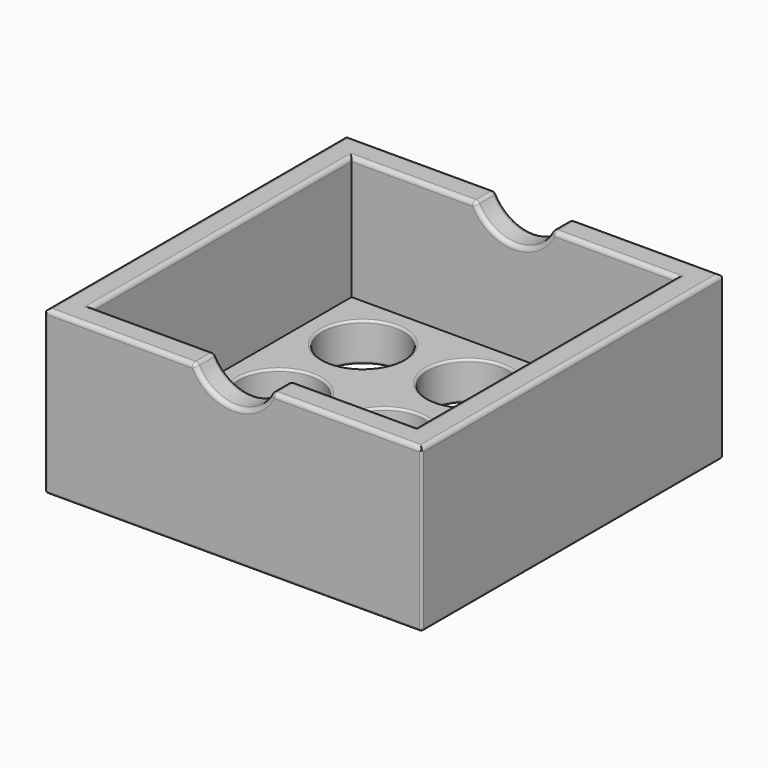
from build123d import *

# Parameters (mm, degrees)
F0_W         = 74
F0_H         = 74
F1_DEPTH     = 37
F0_R         = 9.25
F2_DEPTH     = 8.8
F3_R         = 9.6387493407
F4_DEPTH     = 800
F5_R         = 1
F6_T1_DEPTH  = 36.75
F6_T3_DEPTH  = 85
F6_T5_DEPTH  = 85
F6_S9_W      = 0.51
F6_S9_H      = 0.51
F6_T10_DEPTH = 0.51
F6_S15_W     = 0.51
F6_S15_H     = 0.51
F6_T16_DEPTH = 0.51
F6_S21_W     = 0.51
F6_S21_H     = 0.51
F6_T22_DEPTH = 0.51
F6_S27_W     = 0.51
F6_S27_H     = 0.51
F6_T28_DEPTH = 0.51
F7_R         = 0.5


# Not quite as in the source:
# - a fillet or chamfer that OpenCascade refuses, or shapes differently, is made with other operations: its cross-section is extruded or revolved along the edge and cut away or added


with BuildPart() as f1:
    # F0 (on Top) → F1 (new body)
    with BuildSketch(Plane.XY):
        Polygon((-6, 80), (-6, 0), (-6, -6), (80, -6), (80, 80), align=None)
        with Locations((37, 37)):
            Rectangle(F0_W, F0_H, mode=Mode.SUBTRACT)
    extrude(amount=F1_DEPTH)

    # F0 (on Top) → F2 (join)
    with BuildSketch(Plane.XY):
        with Locations((37, 37)):
            Rectangle(F0_W, F0_H)
        with Locations((13, 13)):
            Circle(F0_R, mode=Mode.SUBTRACT)
        with Locations((37, 13)):
            Circle(F0_R, mode=Mode.SUBTRACT)
        with Locations((61, 13)):
            Circle(F0_R, mode=Mode.SUBTRACT)
        with Locations((13, 37)):
            Circle(F0_R, mode=Mode.SUBTRACT)
        with Locations((13, 61)):
            Circle(F0_R, mode=Mode.SUBTRACT)
        with Locations((37, 37)):
            Circle(F0_R, mode=Mode.SUBTRACT)
        with Locations((61, 37)):
            Circle(F0_R, mode=Mode.SUBTRACT)
        with Locations((37, 61)):
            Circle(F0_R, mode=Mode.SUBTRACT)
        with Locations((61, 61)):
            Circle(F0_R, mode=Mode.SUBTRACT)
    extrude(amount=F2_DEPTH)

    # F3 (on face) → F4 (cut)
    with BuildSketch(Plane.XZ.offset(6)):
        with Locations((37, 41)):
            Circle(F3_R)
    extrude(amount=-F4_DEPTH, mode=Mode.SUBTRACT)

    # F5
    f5_edges = [f1.edges().sort_by_distance(p)[0] for p in [
        (-6, 37, 37),
        (11.115211, 80, 37),
        (28.230423, 77, 37),
        (14.115211, 74, 37),
        (0, 37, 37),
        (14.115211, 0, 37),
        (28.230423, -3, 37),
        (11.115211, -6, 37),
        (62.884789, -6, 37),
        (45.769577, -3, 37),
        (59.884789, 0, 37),
        (74, 37, 37),
        (59.884789, 74, 37),
        (45.769577, 77, 37),
        (62.884789, 80, 37),
        (80, 37, 37),
        (37, -6, 31.361251),
        (37, 0, 31.361251),
        (37, 74, 31.361251),
        (37, 80, 31.361251),
    ]]
    fillet(f5_edges, radius=F5_R)

    # F6: fillet of radius 0.5 on 16 edges, made by hand

    # F6_s2 → F6_t1 (cut)
    with BuildSketch(Plane.XY.offset(0.5)):
        with BuildLine():
            ThreePointArc((79.5, -6), (79.8535533906, -5.8535533906), (80, -5.5))
            Line((80, -5.5), (80, -6))
            Line((80, -6), (79.5, -6))
        make_face()
        with BuildLine():
            ThreePointArc((-6, -5.5), (-5.8535533906, -5.8535533906), (-5.5, -6))
            Line((-5.5, -6), (-6, -6))
            Line((-6, -6), (-6, -5.5))
        make_face()
        with BuildLine():
            ThreePointArc((79.5, 80), (79.8535533906, 79.8535533906), (80, 79.5))
            Line((80, 79.5), (80, 80))
            Line((80, 80), (79.5, 80))
        make_face()
        with BuildLine():
            ThreePointArc((-6, 79.5), (-5.8535533906, 79.8535533906), (-5.5, 80))
            Line((-5.5, 80), (-6, 80))
            Line((-6, 80), (-6, 79.5))
        make_face()
    extrude(amount=F6_T1_DEPTH, mode=Mode.SUBTRACT)

    # F6_s4 → F6_t3 (cut)
    with BuildSketch(Plane.YZ.offset(-5.5)):
        with BuildLine():
            ThreePointArc((-5.5, 0), (-5.8535533906, 0.1464466094), (-6, 0.5))
            Line((-6, 0.5), (-6, 0))
            Line((-6, 0), (-5.5, 0))
        make_face()
        with BuildLine():
            ThreePointArc((80, 0.5), (79.8535533906, 0.1464466094), (79.5, 0))
            Line((79.5, 0), (80, 0))
            Line((80, 0), (80, 0.5))
        make_face()
    extrude(amount=F6_T3_DEPTH, mode=Mode.SUBTRACT)

    # F6_s6 → F6_t5 (cut)
    with BuildSketch(Plane.XZ.offset(-79.5)):
        with BuildLine():
            ThreePointArc((79.5, 0), (79.8535533906, 0.1464466094), (80, 0.5))
            Line((80, 0.5), (80, 0))
            Line((80, 0), (79.5, 0))
        make_face()
        with BuildLine():
            ThreePointArc((-6, 0.5), (-5.8535533906, 0.1464466094), (-5.5, 0))
            Line((-5.5, 0), (-6, 0))
            Line((-6, 0), (-6, 0.5))
        make_face()
    extrude(amount=F6_T5_DEPTH, mode=Mode.SUBTRACT)


with BuildPart() as f6_tool8:
    # F6_s9 → F6_t10 (new body)
    with BuildSketch(Plane.XY.offset(0.5)):
        with Locations((79.755, -5.755)):
            Rectangle(F6_S9_W, F6_S9_H)
    extrude(amount=-F6_T10_DEPTH)

    # F6_s11 → F6_t12 (revolve, cut)
    with BuildSketch(Plane(origin=(79.5, -5.5, 0.5), x_dir=(-0.7071067812, 0.7071067812, 0), z_dir=(-0.7071067812, -0.7071067812, 0))):
        with BuildLine():
            ThreePointArc((0, -0.5), (0.5, 0), (0, 0.5))
            Line((0, 0.5), (0, -0.5))
        make_face()
    revolve(axis=Axis((79.5, -5.5, 0.5), (0, 0, -1)), mode=Mode.SUBTRACT)


with BuildPart() as f1_1:
    add(f1.part)

    # F6_t7: cut F6_tool8
    add(f6_tool8.part, mode=Mode.SUBTRACT)


with BuildPart() as f6_tool14:
    # F6_s15 → F6_t16 (new body)
    with BuildSketch(Plane.YZ.offset(-5.5)):
        with Locations((-5.755, 0.245)):
            Rectangle(F6_S15_W, F6_S15_H)
    extrude(amount=-F6_T16_DEPTH)

    # F6_s17 → F6_t18 (revolve, cut)
    with BuildSketch(Plane(origin=(-5.5, -5.5, 0.5), x_dir=(0, 0.7071067812, 0.7071067812), z_dir=(0, -0.7071067812, 0.7071067812))):
        with BuildLine():
            ThreePointArc((0, -0.5), (0.5, 0), (0, 0.5))
            Line((0, 0.5), (0, -0.5))
        make_face()
    revolve(axis=Axis((-5.5, -5.5, 0.5), (-1, 0, 0)), mode=Mode.SUBTRACT)


with BuildPart() as f1_2:
    add(f1_1.part)

    # F6_t13: cut F6_tool14
    add(f6_tool14.part, mode=Mode.SUBTRACT)


with BuildPart() as f6_tool20:
    # F6_s21 → F6_t22 (new body)
    with BuildSketch(Plane.XZ.offset(-79.5)):
        with Locations((79.755, 0.245)):
            Rectangle(F6_S21_W, F6_S21_H)
    extrude(amount=-F6_T22_DEPTH)

    # F6_s23 → F6_t24 (revolve, cut)
    with BuildSketch(Plane(origin=(79.5, 79.5, 0.5), x_dir=(-0.7071067812, 0, 0.7071067812), z_dir=(-0.7071067812, 0, -0.7071067812))):
        with BuildLine():
            ThreePointArc((0, -0.5), (0.5, 0), (0, 0.5))
            Line((0, 0.5), (0, -0.5))
        make_face()
    revolve(axis=Axis((79.5, 79.5, 0.5), (0, 1, 0)), mode=Mode.SUBTRACT)


with BuildPart() as f1_3:
    add(f1_2.part)

    # F6_t19: cut F6_tool20
    add(f6_tool20.part, mode=Mode.SUBTRACT)


with BuildPart() as f6_tool26:
    # F6_s27 → F6_t28 (new body)
    with BuildSketch(Plane.YZ.offset(-5.5)):
        with Locations((79.755, 0.245)):
            Rectangle(F6_S27_W, F6_S27_H)
    extrude(amount=-F6_T28_DEPTH)

    # F6_s29 → F6_t30 (revolve, cut)
    with BuildSketch(Plane(origin=(-5.5, 79.5, 0.5), x_dir=(0, -0.7071067812, 0.7071067812), z_dir=(0, -0.7071067812, -0.7071067812))):
        with BuildLine():
            ThreePointArc((0, -0.5), (0.5, 0), (0, 0.5))
            Line((0, 0.5), (0, -0.5))
        make_face()
    revolve(axis=Axis((-5.5, 79.5, 0.5), (-1, 0, 0)), mode=Mode.SUBTRACT)


with BuildPart() as f1_4:
    add(f1_3.part)

    # F6_t25: cut F6_tool26
    add(f6_tool26.part, mode=Mode.SUBTRACT)

    # F7
    f7_edges = [f1_4.edges().sort_by_distance(p)[0] for p in [
        (70.25, 13, 4.4),
        (51.75, 13, 0),
        (51.75, 13, 8.8),
        (70.25, 37, 4.4),
        (51.75, 37, 0),
        (51.75, 37, 8.8),
        (70.25, 61, 4.4),
        (51.75, 61, 0),
        (51.75, 61, 8.8),
        (46.25, 61, 4.4),
        (27.75, 61, 0),
        (27.75, 61, 8.8),
        (46.25, 37, 4.4),
        (27.75, 37, 0),
        (27.75, 37, 8.8),
        (46.25, 13, 4.4),
        (27.75, 13, 0),
        (27.75, 13, 8.8),
        (22.25, 13, 4.4),
        (3.75, 13, 0),
        (3.75, 13, 8.8),
        (22.25, 37, 4.4),
        (3.75, 37, 0),
        (3.75, 37, 8.8),
        (22.25, 61, 4.4),
        (3.75, 61, 0),
        (3.75, 61, 8.8),
    ]]
    fillet(f7_edges, radius=F7_R)


solid = f1_4.part
